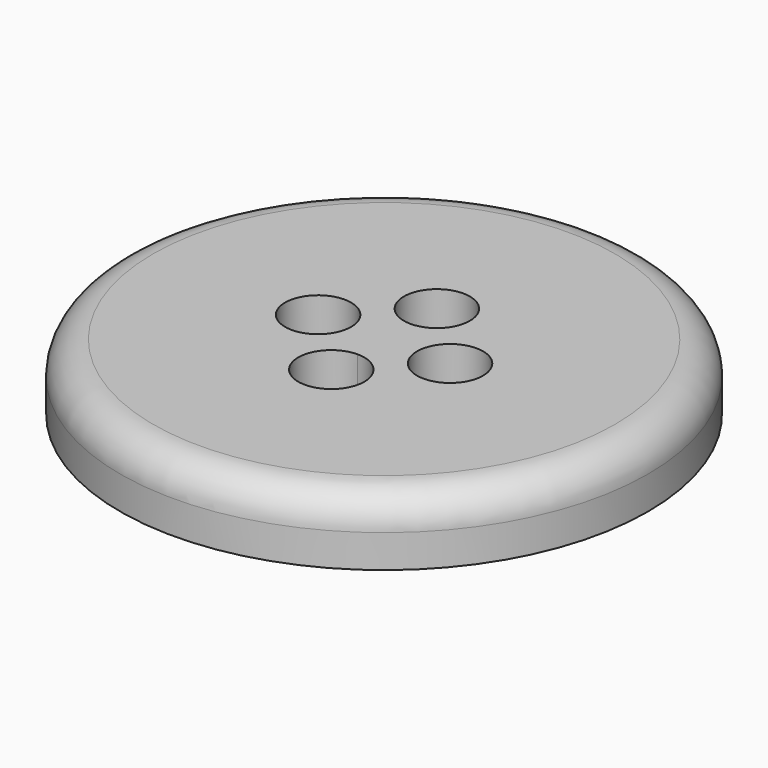
from build123d import *

# Parameters (mm, degrees)
F0_R     = 20
F1_DEPTH = 5
F2_R     = 2.5
F3_R     = 2.5
F4_DEPTH = 25
F5_R     = 6
F6_DEPTH = 2


# Not quite as in the source:
# - a feature names something its author has since deleted; it is built from what else it names


with BuildPart() as f1:
    # F0 (on Top) → F1 (new body)
    with BuildSketch(Plane.XY):
        Circle(F0_R)
    extrude(amount=F1_DEPTH)

    # F2
    f2_edges = [f1.edges().sort_by_distance(p)[0] for p in [
        (-20, 0, 5),
    ]]
    fillet(f2_edges, radius=F2_R)

    # F3 (on Top) → F4 (cut)
    with BuildSketch(Plane.XY):
        with BuildLine():
            ThreePointArc((2.5, 5), (-1.767766953, 6.767766953), (0, 2.5))
            ThreePointArc((0, 2.5), (1.767766953, 3.232233047), (2.5, 5))
        make_face()
        with Locations((-5, 0)):
            Circle(F3_R)
        with BuildLine():
            ThreePointArc((2.5, -5), (1.767766953, -3.232233047), (0, -2.5))
            ThreePointArc((0, -2.5), (-1.767766953, -6.767766953), (2.5, -5))
        make_face()
        with BuildLine():
            ThreePointArc((7.5, 0), (5, 2.5), (2.5, 0))
            ThreePointArc((2.5, 0), (5, -2.5), (7.5, 0))
        make_face()
    extrude(amount=F4_DEPTH, mode=Mode.SUBTRACT)

    # F5 (on Top) → F6 (cut)
    with BuildSketch(Plane.XY):
        Circle(F5_R)
    extrude(amount=F6_DEPTH, mode=Mode.SUBTRACT)


solid = f1.part
